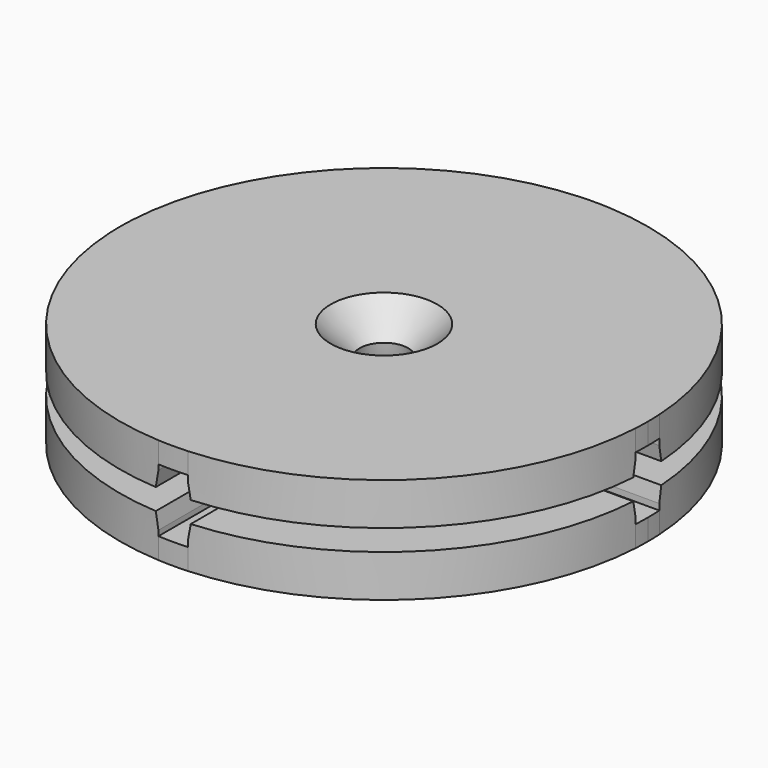
from build123d import *
from build123d import SkipClean  # not in build123d's __all__

# Parameters (mm, degrees)
F0_R         = 2.25
F1_DEPTH     = 2
F2_DEPTH     = 4
F3_SIZE2     = 1.4178204549
F3_SIZE      = 0.25
F3_2_SIZE2   = 1.4178204549
F3_2_SIZE    = 0.25
F3_3_SIZE2   = 1.4178204549
F3_3_SIZE    = 0.25
F3_4_SIZE2   = 1.4178204549
F3_4_SIZE    = 0.25
F4_C1_SIZE2  = 0.2644904711
F4_C1_SIZE   = 1.5
F4_C2_SIZE2  = 0.2644904711
F4_C2_SIZE   = 1.5
F4_C3_SIZE2  = 0.2644904711
F4_C3_SIZE   = 1.5
F4_C4_SIZE2  = 0.2644904711
F4_C4_SIZE   = 1.5
F4_C5_SIZE2  = 0.2644904711
F4_C5_SIZE   = 1.5
F4_C6_SIZE2  = 0.2644904711
F4_C6_SIZE   = 1.5
F4_C7_SIZE2  = 0.2644904711
F4_C7_SIZE   = 1.5
F4_C8_SIZE2  = 0.2644904711
F4_C8_SIZE   = 1.5
F4_C9_SIZE2  = 0.2644904711
F4_C9_SIZE   = 1.5
F4_C10_SIZE2 = 0.2644904711
F4_C10_SIZE  = 1.5
F4_C11_SIZE2 = 1.5
F4_C11_SIZE  = 0.2644904711


# Not quite as in the source:
# - a fillet or chamfer that OpenCascade refuses, or shapes differently, is made with other operations: its cross-section is extruded or revolved along the edge and cut away or added


with BuildPart() as f1:
    # F0 (on Top) → F1 (new body)
    with BuildSketch(Plane.XY):
        with BuildLine():
            ThreePointArc((15.9888242219, -1.4), (16.0346987618, -0.7006679805), (16.05, 0))
            ThreePointArc((16.05, 0), (16.0346987618, 0.7006679805), (15.9888242219, 1.4))
            ThreePointArc((15.9888242219, 1.4), (11.349063838, 11.349063838), (1.4, 15.9888242219))
            ThreePointArc((1.4, 15.9888242219), (0, 16.05), (-1.4, 15.9888242219))
            ThreePointArc((-1.4, 15.9888242219), (-11.349063838, 11.349063838), (-15.9888242219, 1.4))
            ThreePointArc((-15.9888242219, 1.4), (-16.05, 0), (-15.9888242219, -1.4))
            ThreePointArc((-15.9888242219, -1.4), (-11.349063838, -11.349063838), (-1.4, -15.9888242219))
            ThreePointArc((-1.4, -15.9888242219), (0, -16.05), (1.4, -15.9888242219))
            ThreePointArc((1.4, -15.9888242219), (11.349063838, -11.349063838), (15.9888242219, -1.4))
        make_face()
        with BuildLine():
            ThreePointArc((5.0199601592, 4.95), (6.5227762158, 2.6750496143), (7.05, 0))
            ThreePointArc((7.05, 0), (-2.6750496143, -6.5227762158), (-5.0199601592, 4.95))
            ThreePointArc((-5.0199601592, 4.95), (0, 7.05), (5.0199601592, 4.95))
        make_face(mode=Mode.SUBTRACT)
        with BuildLine():
            ThreePointArc((-5.0199601592, 4.95), (-2.6750496143, -6.5227762158), (7.05, 0))
            ThreePointArc((7.05, 0), (6.5227762158, 2.6750496143), (5.0199601592, 4.95))
            Line((5.0199601592, 4.95), (-5.0199601592, 4.95))
        make_face()
        Circle(F0_R, mode=Mode.SUBTRACT)
        with BuildLine():
            Line((-5.0199601592, 4.95), (5.0199601592, 4.95))
            ThreePointArc((5.0199601592, 4.95), (0, 7.05), (-5.0199601592, 4.95))
        make_face()
        with BuildLine():
            ThreePointArc((1.4, 15.9888242219), (11.349063838, 11.349063838), (15.9888242219, 1.4))
            Line((15.9888242219, 1.4), (24.9607692189, 1.4))
            ThreePointArc((24.9607692189, 1.4), (17.6776695297, 17.6776695297), (1.4, 24.9607692189))
            Line((1.4, 24.9607692189), (1.4, 15.9888242219))
        make_face()
        with BuildLine():
            ThreePointArc((-15.9888242219, 1.4), (-11.349063838, 11.349063838), (-1.4, 15.9888242219))
            Line((-1.4, 15.9888242219), (-1.4, 24.9607692189))
            ThreePointArc((-1.4, 24.9607692189), (-17.6776695297, 17.6776695297), (-24.9607692189, 1.4))
            Line((-24.9607692189, 1.4), (-15.9888242219, 1.4))
        make_face()
        with BuildLine():
            ThreePointArc((-1.4, 15.9888242219), (0, 16.05), (1.4, 15.9888242219))
            Line((1.4, 15.9888242219), (1.4, 24.9607692189))
            ThreePointArc((1.4, 24.9607692189), (0, 25), (-1.4, 24.9607692189))
            Line((-1.4, 24.9607692189), (-1.4, 15.9888242219))
        make_face()
        with BuildLine():
            ThreePointArc((-15.9888242219, -1.4), (-16.05, 0), (-15.9888242219, 1.4))
            Line((-15.9888242219, 1.4), (-24.9607692189, 1.4))
            ThreePointArc((-24.9607692189, 1.4), (-25, 0), (-24.9607692189, -1.4))
            Line((-24.9607692189, -1.4), (-15.9888242219, -1.4))
        make_face()
        with BuildLine():
            Line((-1.4, -24.9607692189), (-1.4, -15.9888242219))
            ThreePointArc((-1.4, -15.9888242219), (-11.349063838, -11.349063838), (-15.9888242219, -1.4))
            Line((-15.9888242219, -1.4), (-24.9607692189, -1.4))
            ThreePointArc((-24.9607692189, -1.4), (-17.6776695297, -17.6776695297), (-1.4, -24.9607692189))
        make_face()
        with BuildLine():
            Line((1.4, -24.9607692189), (1.4, -15.9888242219))
            ThreePointArc((1.4, -15.9888242219), (0, -16.05), (-1.4, -15.9888242219))
            Line((-1.4, -15.9888242219), (-1.4, -24.9607692189))
            ThreePointArc((-1.4, -24.9607692189), (0, -25), (1.4, -24.9607692189))
        make_face()
        with BuildLine():
            Line((24.9607692189, -1.4), (15.9888242219, -1.4))
            ThreePointArc((15.9888242219, -1.4), (11.349063838, -11.349063838), (1.4, -15.9888242219))
            Line((1.4, -15.9888242219), (1.4, -24.9607692189))
            ThreePointArc((1.4, -24.9607692189), (17.6776695297, -17.6776695297), (24.9607692189, -1.4))
        make_face()
        with BuildLine():
            ThreePointArc((15.9888242219, 1.4), (16.0346987618, 0.7006679805), (16.05, 0))
            ThreePointArc((16.05, 0), (16.0346987618, -0.7006679805), (15.9888242219, -1.4))
            Line((15.9888242219, -1.4), (24.9607692189, -1.4))
            ThreePointArc((24.9607692189, -1.4), (24.9901903802, -0.7002747772), (25, 0))
            ThreePointArc((25, 0), (24.9901903802, 0.7002747772), (24.9607692189, 1.4))
            Line((24.9607692189, 1.4), (15.9888242219, 1.4))
        make_face()
    extrude(amount=F1_DEPTH)

    # F0 (on Top) → F2 (join)
    with BuildSketch(Plane.XY):
        with BuildLine():
            ThreePointArc((-5.0199601592, 4.95), (-2.6750496143, -6.5227762158), (7.05, 0))
            ThreePointArc((7.05, 0), (6.5227762158, 2.6750496143), (5.0199601592, 4.95))
            Line((5.0199601592, 4.95), (-5.0199601592, 4.95))
        make_face()
        Circle(F0_R, mode=Mode.SUBTRACT)
        with BuildLine():
            Line((24.9607692189, -1.4), (15.9888242219, -1.4))
            ThreePointArc((15.9888242219, -1.4), (11.349063838, -11.349063838), (1.4, -15.9888242219))
            Line((1.4, -15.9888242219), (1.4, -24.9607692189))
            ThreePointArc((1.4, -24.9607692189), (17.6776695297, -17.6776695297), (24.9607692189, -1.4))
        make_face()
        with BuildLine():
            Line((-1.4, -24.9607692189), (-1.4, -15.9888242219))
            ThreePointArc((-1.4, -15.9888242219), (-11.349063838, -11.349063838), (-15.9888242219, -1.4))
            Line((-15.9888242219, -1.4), (-24.9607692189, -1.4))
            ThreePointArc((-24.9607692189, -1.4), (-17.6776695297, -17.6776695297), (-1.4, -24.9607692189))
        make_face()
        with BuildLine():
            ThreePointArc((-15.9888242219, 1.4), (-11.349063838, 11.349063838), (-1.4, 15.9888242219))
            Line((-1.4, 15.9888242219), (-1.4, 24.9607692189))
            ThreePointArc((-1.4, 24.9607692189), (-17.6776695297, 17.6776695297), (-24.9607692189, 1.4))
            Line((-24.9607692189, 1.4), (-15.9888242219, 1.4))
        make_face()
        with BuildLine():
            ThreePointArc((1.4, 15.9888242219), (11.349063838, 11.349063838), (15.9888242219, 1.4))
            Line((15.9888242219, 1.4), (24.9607692189, 1.4))
            ThreePointArc((24.9607692189, 1.4), (17.6776695297, 17.6776695297), (1.4, 24.9607692189))
            Line((1.4, 24.9607692189), (1.4, 15.9888242219))
        make_face()
    with SkipClean():  # cleaning this boolean's faces spoils the solid; the shape is the same uncleaned
        extrude(amount=F2_DEPTH)

    # F3
    f3_edges = [f1.edges().sort_by_distance(p)[0] for p in [
        (-20.474797, -1.4, 4),
    ]]
    f3_side = f1.faces().sort_by_distance((-13.527768, -13.527768, 4))[0]
    chamfer(f3_edges, length=F3_SIZE, length2=F3_SIZE2, reference=f3_side)

    # F3#2
    f3_2_edges = [f1.edges().sort_by_distance(p)[0] for p in [
        (20.474797, 1.4, 4),
    ]]
    f3_2_side = f1.faces().sort_by_distance((13.527768, 13.527768, 4))[0]
    chamfer(f3_2_edges, length=F3_2_SIZE, length2=F3_2_SIZE2, reference=f3_2_side)

    # F3#3
    f3_3_edges = [f1.edges().sort_by_distance(p)[0] for p in [
        (0, -7.05, 4),
    ]]
    f3_3_side = f1.faces().sort_by_distance((0, -6.864849, 4))[0]
    chamfer(f3_3_edges, length=F3_3_SIZE, length2=F3_3_SIZE2, reference=f3_3_side)

    # F3#4
    f3_4_edges = [f1.edges().sort_by_distance(p)[0] for p in [
        (1.4, -20.474797, 4),
    ]]
    f3_4_side = f1.faces().sort_by_distance((13.527768, -13.527768, 4))[0]
    chamfer(f3_4_edges, length=F3_4_SIZE, length2=F3_4_SIZE2, reference=f3_4_side)

    # F4: chamfer of 1.5 x 0.2644904711 on 11 edges, made by hand

    # F4_c1
    f4_c1_edges = [f1.edges().sort_by_distance(p)[0] for p in [
        (11.4375065831, -11.2599264279, 4),
    ]]
    f4_c1_side = f1.faces().sort_by_distance((11.4375065831, -11.2599264279, 3.9947101906))[0]
    chamfer(f4_c1_edges, length=F4_C1_SIZE, length2=F4_C1_SIZE2, reference=f4_c1_side)

    # F4_c2
    f4_c2_edges = [f1.edges().sort_by_distance(p)[0] for p in [
        (20.607539698, -1.4, 4),
    ]]
    f4_c2_side = f1.faces().sort_by_distance((20.607539698, -1.4, 3.9947101906))[0]
    chamfer(f4_c2_edges, length=F4_C2_SIZE, length2=F4_C2_SIZE2, reference=f4_c2_side)

    # F4_c3
    f4_c3_edges = [f1.edges().sort_by_distance(p)[0] for p in [
        (-1.4, -20.4747967204, 4),
    ]]
    f4_c3_side = f1.faces().sort_by_distance((-1.4, -20.4747967204, 3.9947101906))[0]
    chamfer(f4_c3_edges, length=F4_C3_SIZE, length2=F4_C3_SIZE2, reference=f4_c3_side)

    # F4_c4
    f4_c4_edges = [f1.edges().sort_by_distance(p)[0] for p in [
        (-11.3542133554, -11.3439119831, 4),
    ]]
    f4_c4_side = f1.faces().sort_by_distance((-11.3542133554, -11.3439119831, 3.9947101906))[0]
    chamfer(f4_c4_edges, length=F4_C4_SIZE, length2=F4_C4_SIZE2, reference=f4_c4_side)

    # F4_c5
    f4_c5_edges = [f1.edges().sort_by_distance(p)[0] for p in [
        (-20.4747967204, 1.4, 4),
    ]]
    f4_c5_side = f1.faces().sort_by_distance((-20.4747967204, 1.4, 3.9947101906))[0]
    chamfer(f4_c5_edges, length=F4_C5_SIZE, length2=F4_C5_SIZE2, reference=f4_c5_side)

    # F4_c6
    f4_c6_edges = [f1.edges().sort_by_distance(p)[0] for p in [
        (-11.2547344431, 11.442615637, 4),
    ]]
    f4_c6_side = f1.faces().sort_by_distance((-11.2547344431, 11.442615637, 3.9947101906))[0]
    chamfer(f4_c6_edges, length=F4_C6_SIZE, length2=F4_C6_SIZE2, reference=f4_c6_side)

    # F4_c7
    f4_c7_edges = [f1.edges().sort_by_distance(p)[0] for p in [
        (-1.4, 20.607539698, 4),
    ]]
    f4_c7_side = f1.faces().sort_by_distance((-1.4, 20.607539698, 3.9947101906))[0]
    chamfer(f4_c7_edges, length=F4_C7_SIZE, length2=F4_C7_SIZE2, reference=f4_c7_side)

    # F4_c8
    f4_c8_edges = [f1.edges().sort_by_distance(p)[0] for p in [
        (1.4, 20.4747967204, 4),
    ]]
    f4_c8_side = f1.faces().sort_by_distance((1.4, 20.4747967204, 3.9947101906))[0]
    chamfer(f4_c8_edges, length=F4_C8_SIZE, length2=F4_C8_SIZE2, reference=f4_c8_side)

    # F4_c9
    f4_c9_edges = [f1.edges().sort_by_distance(p)[0] for p in [
        (11.3542133554, 11.3439119831, 4),
    ]]
    f4_c9_side = f1.faces().sort_by_distance((11.3542133554, 11.3439119831, 3.9947101906))[0]
    chamfer(f4_c9_edges, length=F4_C9_SIZE, length2=F4_C9_SIZE2, reference=f4_c9_side)

    # F4_c10
    f4_c10_edges = [f1.edges().sort_by_distance(p)[0] for p in [
        (0, 4.95, 4),
    ]]
    f4_c10_side = f1.faces().sort_by_distance((0, 4.95, 3.9947101906))[0]
    chamfer(f4_c10_edges, length=F4_C10_SIZE, length2=F4_C10_SIZE2, reference=f4_c10_side)

    # F4_c11
    f4_c11_edges = [f1.edges().sort_by_distance(p)[0] for p in [
        (-2.25, 0, 4),
    ]]
    f4_c11_side = f1.faces().sort_by_distance((-2.2552898094, 0, 4))[0]
    chamfer(f4_c11_edges, length=F4_C11_SIZE, length2=F4_C11_SIZE2, reference=f4_c11_side)


with BuildPart() as f5_1:
    # F5: instance of F1
    add(f1.part.mirror(Plane.XY), clean=False)


with BuildPart() as f5_1_1:
    # F6: moved
    add(f5_1.part.moved(Location((0, 0, 10))), clean=False)

    # F7: chamfer of 2.8 on 1 edges, made by hand

    # F7_s1 → F7_t2 (revolve, cut)
    with BuildSketch(Plane.XZ):
        Polygon((2.25, 7.2), (5.05, 10), (2.25, 10), align=None)
    revolve(axis=Axis((0, 0, 10), (0, 0, 1)), mode=Mode.SUBTRACT)


solid = Compound([f1.part, f5_1_1.part])
